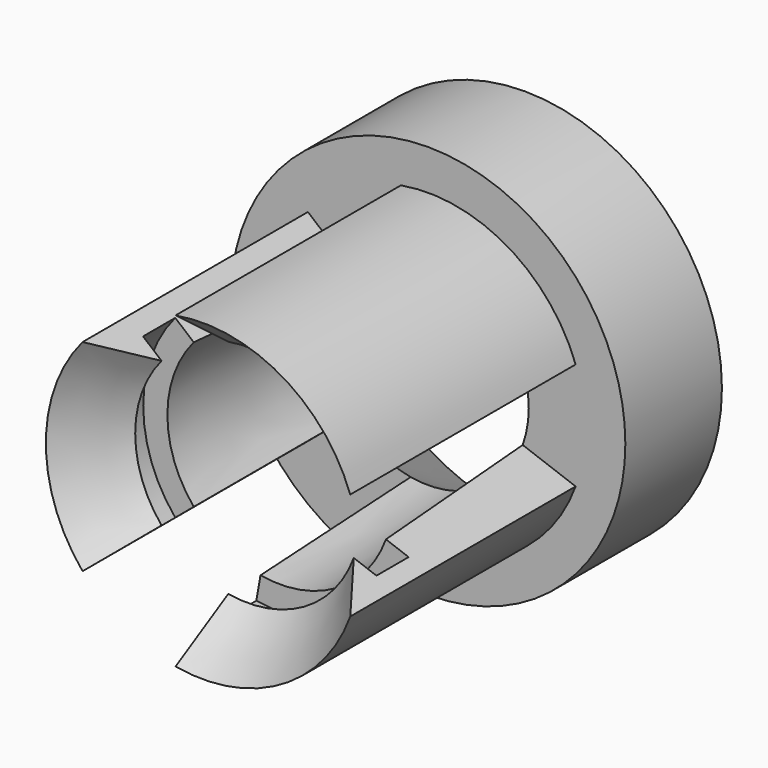
from build123d import *

# Parameters (mm, degrees)
F3_DEPTH = 10


with BuildPart() as f1:
    # F0 (on Right) → F1 (revolve)
    with BuildSketch(Plane.YZ):
        Polygon((-7.6, 2.8), (-3, 2.5), (0, 4.4), (0, 4.9), (-3, 4.9), (-3, 3.9), (-10, 3.9), (-8.6, 2.8), (-8.6, 3.4), (-7.6, 3.4), align=None)
    revolve(axis=Axis((0, -6.9740121253, 0), (0, -1, 0)))

    # F2 (on face) → F3 (cut)
    with BuildSketch(Plane.XZ.offset(3)):
        with BuildLine():
            Line((-2.9875733282, 2.5068716778), (0, 0))
            Line((0, 0), (-0.6772278929, 3.8407502367))
            ThreePointArc((-0.6772278929, 3.8407502367), (-1.95, 3.3774990748), (-2.9875733282, 2.5068716778))
        make_face()
        with BuildLine():
            Line((3.6648012211, 1.333878559), (0, 0))
            Line((0, 0), (3.9, 0))
            ThreePointArc((3.9, 0), (3.8407502367, 0.6772278929), (3.6648012211, 1.333878559))
        make_face()
        with BuildLine():
            Line((3.9, 0), (0, 0))
            Line((0, 0), (3.6648012211, -1.333878559))
            ThreePointArc((3.6648012211, -1.333878559), (3.8407502367, -0.6772278929), (3.9, 0))
        make_face()
        with BuildLine():
            Line((-0.6772278929, -3.8407502367), (0, 0))
            Line((0, 0), (-2.9875733282, -2.5068716778))
            ThreePointArc((-2.9875733282, -2.5068716778), (-1.95, -3.3774990748), (-0.6772278929, -3.8407502367))
        make_face()
        with BuildLine():
            Line((-0.8508760706, 4.8255579898), (-0.6772278929, 3.8407502367))
            ThreePointArc((-0.6772278929, 3.8407502367), (1.95, 3.3774990748), (3.6648012211, 1.333878559))
            Line((3.6648012211, 1.333878559), (4.6044938419, 1.6758987023))
            ThreePointArc((4.6044938419, 1.6758987023), (2.45, 4.2435244785), (-0.8508760706, 4.8255579898))
        make_face()
        with BuildLine():
            ThreePointArc((3.6648012211, 1.333878559), (3.8407502367, 0.6772278929), (3.9, 0))
            Line((3.9, 0), (4.9, 0))
            ThreePointArc((4.9, 0), (4.8255579898, 0.8508760706), (4.6044938419, 1.6758987023))
            Line((4.6044938419, 1.6758987023), (3.6648012211, 1.333878559))
        make_face()
        with BuildLine():
            Line((4.9, 0), (3.9, 0))
            ThreePointArc((3.9, 0), (3.8407502367, -0.6772278929), (3.6648012211, -1.333878559))
            Line((3.6648012211, -1.333878559), (4.6044938419, -1.6758987023))
            ThreePointArc((4.6044938419, -1.6758987023), (4.8255579898, -0.8508760706), (4.9, 0))
        make_face()
        with BuildLine():
            ThreePointArc((3.6648012211, -1.333878559), (1.95, -3.3774990748), (-0.6772278929, -3.8407502367))
            Line((-0.6772278929, -3.8407502367), (-0.8508760706, -4.8255579898))
            ThreePointArc((-0.8508760706, -4.8255579898), (2.45, -4.2435244785), (4.6044938419, -1.6758987023))
            Line((4.6044938419, -1.6758987023), (3.6648012211, -1.333878559))
        make_face()
    extrude(amount=F3_DEPTH, mode=Mode.SUBTRACT)


solid = f1.part
